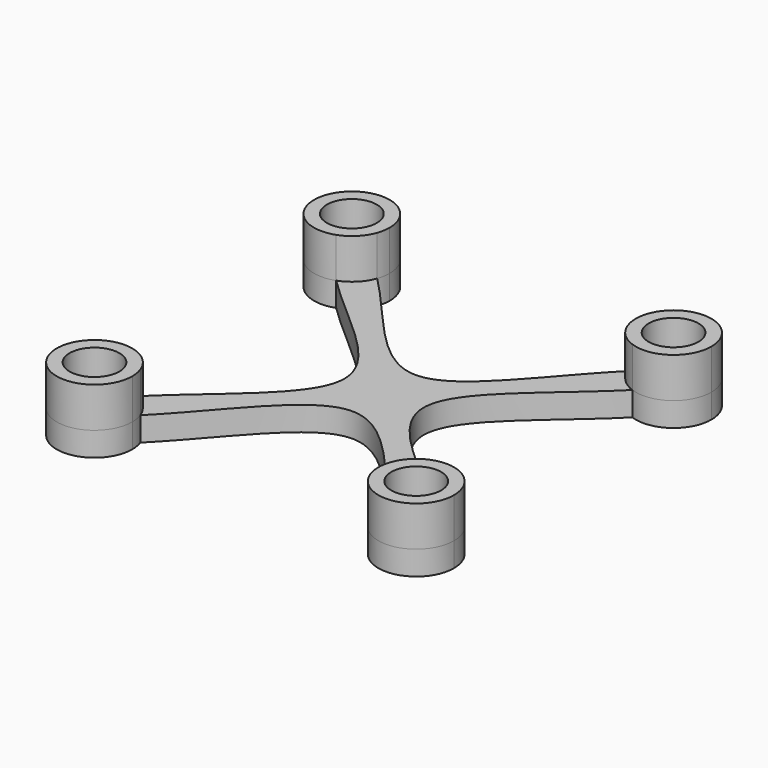
from build123d import *

# Parameters (mm, degrees)
F0_R     = 1.55
F1_DEPTH = 4
F2_DEPTH = 1.5


with BuildPart() as f1:
    # F0 (on Top) → F1 (new body)
    with BuildSketch(Plane.XY):
        with BuildLine():
            ThreePointArc((-7.7891478946, 9.203361457), (-7.6850483323, 9.5956501809), (-7.65, 10))
            ThreePointArc((-7.65, 10), (-11.9228365214, 11.3509995233), (-9.203361457, 7.7891478946))
            ThreePointArc((-9.203361457, 7.7891478946), (-8.3382990642, 8.3382990642), (-7.7891478946, 9.203361457))
        make_face()
        with Locations((-10, 10)):
            Circle(F0_R, mode=Mode.SUBTRACT)
    extrude(amount=F1_DEPTH)


with BuildPart() as f1b:
    # F0 (on Top) → F1, piece 2 (new body)
    with BuildSketch(Plane.XY):
        with BuildLine():
            ThreePointArc((-7.7891478946, -9.203361457), (-8.3382990642, -8.3382990642), (-9.203361457, -7.7891478946))
            ThreePointArc((-9.203361457, -7.7891478946), (-11.9228365214, -11.3509995233), (-7.65, -10))
            ThreePointArc((-7.65, -10), (-7.6850483323, -9.5956501809), (-7.7891478946, -9.203361457))
        make_face()
        with Locations((-10, -10)):
            Circle(F0_R, mode=Mode.SUBTRACT)
    extrude(amount=F1_DEPTH)


with BuildPart() as f1c:
    # F0 (on Top) → F1, piece 3 (new body)
    with BuildSketch(Plane.XY):
        with BuildLine():
            ThreePointArc((12.35, 10), (9.5956501809, 12.3149516677), (7.7891478946, 9.203361457))
            ThreePointArc((7.7891478946, 9.203361457), (8.3382990642, 8.3382990642), (9.203361457, 7.7891478946))
            ThreePointArc((9.203361457, 7.7891478946), (11.3509995233, 8.0771634786), (12.35, 10))
        make_face()
        with Locations((10, 10)):
            Circle(F0_R, mode=Mode.SUBTRACT)
    extrude(amount=F1_DEPTH)


with BuildPart() as f1d:
    # F0 (on Top) → F1, piece 4 (new body)
    with BuildSketch(Plane.XY):
        with BuildLine():
            ThreePointArc((9.203361457, -7.7891478946), (8.3382990642, -8.3382990642), (7.7891478946, -9.203361457))
            ThreePointArc((7.7891478946, -9.203361457), (9.5956501809, -12.3149516677), (12.35, -10))
            ThreePointArc((12.35, -10), (11.3509995233, -8.0771634786), (9.203361457, -7.7891478946))
        make_face()
        with Locations((10, -10)):
            Circle(F0_R, mode=Mode.SUBTRACT)
    extrude(amount=F1_DEPTH)


with BuildPart() as f2:
    # F0 (on Top) → F2 (new body)
    with BuildSketch(Plane.XY):
        with BuildLine():
            ThreePointArc((-7.7891478946, 9.203361457), (-7.6850483323, 9.5956501809), (-7.65, 10))
            ThreePointArc((-7.65, 10), (-11.9228365214, 11.3509995233), (-9.203361457, 7.7891478946))
            ThreePointArc((-9.203361457, 7.7891478946), (-8.3382990642, 8.3382990642), (-7.7891478946, 9.203361457))
        make_face()
        with Locations((-10, 10)):
            Circle(F0_R, mode=Mode.SUBTRACT)
        with BuildLine():
            ThreePointArc((-7.7891478946, 9.203361457), (-8.3382990642, 8.3382990642), (-9.203361457, 7.7891478946))
            add(Edge.make_bspline(
                [(-9.203361457, 7.7891478946), (-6.3624616014, 4.948248039), (1.441069995, -0.0242898241), (-6.3138819532, -4.8996683909), (-9.203361457, -7.7891478946)],
                knots=[0, 0, 0, 0, 0.5, 1, 1, 1, 1], degree=3))
            ThreePointArc((-9.203361457, -7.7891478946), (-8.3382990642, -8.3382990642), (-7.7891478946, -9.203361457))
            add(Edge.make_bspline(
                [(7.7891478946, -9.203361457), (4.948248039, -6.3624616014), (-0.0242898241, 1.441069995), (-4.8996683909, -6.3138819532), (-7.7891478946, -9.203361457)],
                knots=[0, 0, 0, 0, 0.5, 1, 1, 1, 1], degree=3))
            ThreePointArc((7.7891478946, -9.203361457), (8.3382990642, -8.3382990642), (9.203361457, -7.7891478946))
            add(Edge.make_bspline(
                [(9.203361457, -7.7891478946), (6.3624616014, -4.948248039), (-1.441069995, 0.0242898241), (6.3138819532, 4.8996683909), (9.203361457, 7.7891478946)],
                knots=[0, 0, 0, 0, 0.5, 1, 1, 1, 1], degree=3))
            ThreePointArc((9.203361457, 7.7891478946), (8.3382990642, 8.3382990642), (7.7891478946, 9.203361457))
            add(Edge.make_bspline(
                [(-7.7891478946, 9.203361457), (-4.948248039, 6.3624616014), (0.0242898241, -1.441069995), (4.8996683909, 6.3138819532), (7.7891478946, 9.203361457)],
                knots=[0, 0, 0, 0, 0.5, 1, 1, 1, 1], degree=3))
        make_face()
        with BuildLine():
            ThreePointArc((-7.7891478946, -9.203361457), (-8.3382990642, -8.3382990642), (-9.203361457, -7.7891478946))
            ThreePointArc((-9.203361457, -7.7891478946), (-11.9228365214, -11.3509995233), (-7.65, -10))
            ThreePointArc((-7.65, -10), (-7.6850483323, -9.5956501809), (-7.7891478946, -9.203361457))
        make_face()
        with Locations((-10, -10)):
            Circle(F0_R, mode=Mode.SUBTRACT)
        with BuildLine():
            ThreePointArc((12.35, 10), (9.5956501809, 12.3149516677), (7.7891478946, 9.203361457))
            ThreePointArc((7.7891478946, 9.203361457), (8.3382990642, 8.3382990642), (9.203361457, 7.7891478946))
            ThreePointArc((9.203361457, 7.7891478946), (11.3509995233, 8.0771634786), (12.35, 10))
        make_face()
        with Locations((10, 10)):
            Circle(F0_R, mode=Mode.SUBTRACT)
        with BuildLine():
            ThreePointArc((9.203361457, -7.7891478946), (8.3382990642, -8.3382990642), (7.7891478946, -9.203361457))
            ThreePointArc((7.7891478946, -9.203361457), (9.5956501809, -12.3149516677), (12.35, -10))
            ThreePointArc((12.35, -10), (11.3509995233, -8.0771634786), (9.203361457, -7.7891478946))
        make_face()
        with Locations((10, -10)):
            Circle(F0_R, mode=Mode.SUBTRACT)
    extrude(amount=F2_DEPTH)


solid = Compound([f1.part, f1b.part, f1c.part, f1d.part, f2.part])
